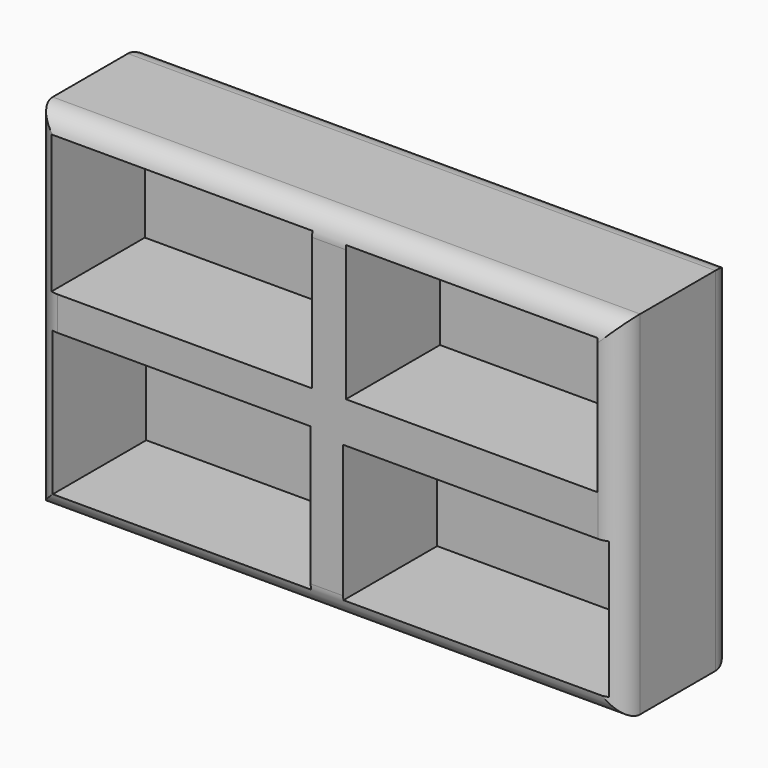
from build123d import *

# Parameters (mm, degrees)
F0_W        = 127
F0_H        = 76.2
F1_DEPTH    = 30.48
F2_W        = 56.4744591247
F2_H        = 29.9161975272
F2_W_2      = 54.3375890702
F2_H_2      = 29.3056648225
F2_W_3      = 57.0849904325
F2_H_3      = 29.6109346673
F2_W_4      = 55.8639247902
F2_H_4      = 31.1372692231
F3_DEPTH    = 25.4
F4_T1_DEPTH = 152.4
F4_T3_DEPTH = 101.6


# Not quite as in the source:
# - a fillet or chamfer that OpenCascade refuses, or shapes differently, is made with other operations: its cross-section is extruded or revolved along the edge and cut away or added


with BuildPart() as f1:
    # F0 (on Front) → F1 (new body)
    with BuildSketch(Plane.XZ):
        Rectangle(F0_W, F0_H)
    extrude(amount=F1_DEPTH)

    # F2 (on face) → F3 (cut)
    with BuildSketch(Plane.XZ.offset(30.48)):
        with Locations((-31.5951720113, 19.2318481859)):
            Rectangle(F2_W, F2_H)
        with Locations((31.1372699216, 19.23184935)):
            Rectangle(F2_W_2, F2_H_2)
        with Locations((31.9004367338, -19.0792032517)):
            Rectangle(F2_W_3, F2_H_3)
        with Locations((-31.5951702651, -18.6213011621)):
            Rectangle(F2_W_4, F2_H_4)
    extrude(amount=-F3_DEPTH, mode=Mode.SUBTRACT)

    # F4: fillet of radius 5.08 on 8 edges, made by hand

    # F4_s2 → F4_t1 (cut)
    with BuildSketch(Plane.YZ.offset(-76.2)):
        with BuildLine():
            ThreePointArc((-25.4, -38.1), (-28.9921024484, -36.6121024484), (-30.48, -33.02))
            Line((-30.48, -33.02), (-30.48, -38.1))
            Line((-30.48, -38.1), (-25.4, -38.1))
        make_face()
        with BuildLine():
            ThreePointArc((-25.4, 38.1), (-28.9921024484, 36.6121024484), (-30.48, 33.02))
            Line((-30.48, 33.02), (-30.48, 38.1))
            Line((-30.48, 38.1), (-25.4, 38.1))
        make_face()
        with BuildLine():
            ThreePointArc((-5.08, -38.1), (-1.4878975516, -36.6121024484), (0, -33.02))
            Line((0, -33.02), (0, -38.1))
            Line((0, -38.1), (-5.08, -38.1))
        make_face()
        with BuildLine():
            ThreePointArc((-5.08, 38.1), (-1.4878975516, 36.6121024484), (0, 33.02))
            Line((0, 33.02), (0, 38.1))
            Line((0, 38.1), (-5.08, 38.1))
        make_face()
    extrude(amount=F4_T1_DEPTH, mode=Mode.SUBTRACT)

    # F4_s4 → F4_t3 (cut)
    with BuildSketch(Plane.XY.offset(-50.8)):
        with BuildLine():
            ThreePointArc((-58.42, -30.48), (-62.0121024484, -28.9921024484), (-63.5, -25.4))
            Line((-63.5, -25.4), (-63.5, -30.48))
            Line((-63.5, -30.48), (-58.42, -30.48))
        make_face()
        with BuildLine():
            ThreePointArc((63.5, -25.4), (62.0121024484, -28.9921024484), (58.42, -30.48))
            Line((58.42, -30.48), (63.5, -30.48))
            Line((63.5, -30.48), (63.5, -25.4))
        make_face()
        with BuildLine():
            ThreePointArc((-58.42, 0), (-62.0121024484, -1.4878975516), (-63.5, -5.08))
            Line((-63.5, -5.08), (-63.5, 0))
            Line((-63.5, 0), (-58.42, 0))
        make_face()
        with BuildLine():
            ThreePointArc((63.5, -5.08), (62.0121024484, -1.4878975516), (58.42, 0))
            Line((58.42, 0), (63.5, 0))
            Line((63.5, 0), (63.5, -5.08))
        make_face()
    extrude(amount=F4_T3_DEPTH, mode=Mode.SUBTRACT)


solid = f1.part
